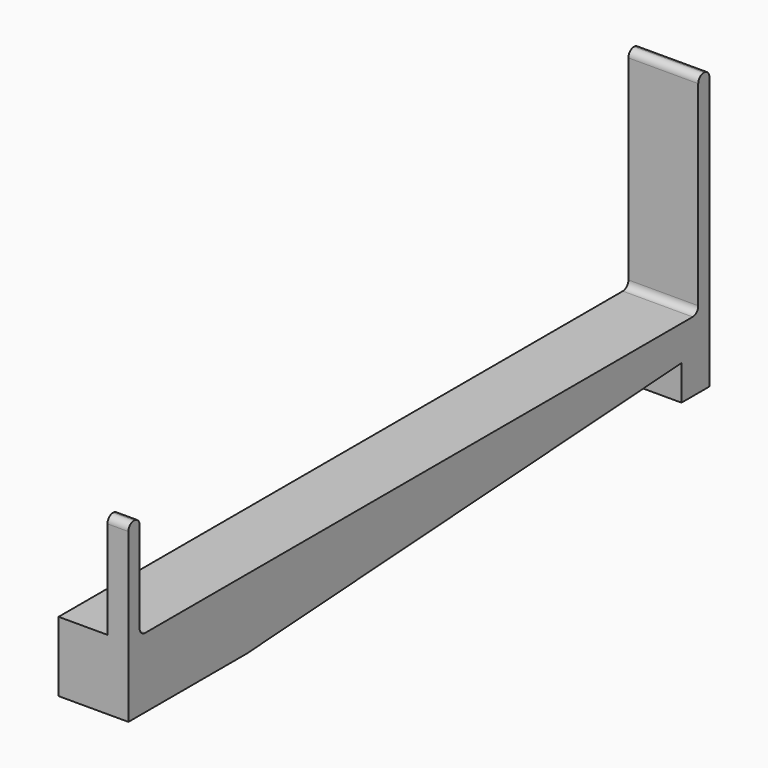
from build123d import *

# Parameters (mm, degrees)
F0_W      = 10
F0_H      = 104
F1_DEPTH  = 10
F2_W      = 10
F2_H      = 2
F3_DEPTH  = 15
F4_W      = 10
F4_H      = 2
F5_DEPTH  = 30
F7_DEPTH  = 10.001
F8_R      = 0.99999
F9_W      = 3
F9_H      = 15
F10_DEPTH = 7


# Not quite as in the source:
# - a fillet or chamfer is up to 0.001 mm smaller than in the source, because OpenCascade refuses the exact size


with BuildPart() as f1:
    # F0 (on Top) → F1 (new body)
    with BuildSketch(Plane.XY):
        Rectangle(F0_W, F0_H)
    extrude(amount=F1_DEPTH)

    # F2 (on face) → F3 (join)
    with BuildSketch(Plane.XY.offset(10)):
        with Locations((0, -51)):
            Rectangle(F2_W, F2_H)
    extrude(amount=F3_DEPTH)

    # F4 (on face) → F5 (join)
    with BuildSketch(Plane.XY.offset(10)):
        with Locations((0, 51)):
            Rectangle(F4_W, F4_H)
    extrude(amount=F5_DEPTH)

    # F6 (on face) → F7 (cut, through all)
    with BuildSketch(Plane.YZ.offset(5)):
        Polygon((47, 5), (-30.8395786217, 0), (47, 0), align=None)
    extrude(amount=-F7_DEPTH, mode=Mode.SUBTRACT)

    # F8 (radius 1 in the source; OpenCascade refuses exactly that, so slightly less here)
    f8_edges = [f1.edges().sort_by_distance(p)[0] for p in [
        (0, 50, 40),
        (0, 52, 40),
        (0, -52, 25),
        (0, -50, 25),
        (0, 50, 10),
        (0, -50, 10),
    ]]
    fillet(f8_edges, radius=F8_R)

    # F9 (on face) → F10 (cut)
    with BuildSketch(Plane(origin=(-5, 0, 0), x_dir=(0, -1, 0), z_dir=(-1, 0, 0))):
        with Locations((50.5, 17.5)):
            Rectangle(F9_W, F9_H)
    extrude(amount=-F10_DEPTH, mode=Mode.SUBTRACT)


solid = f1.part
